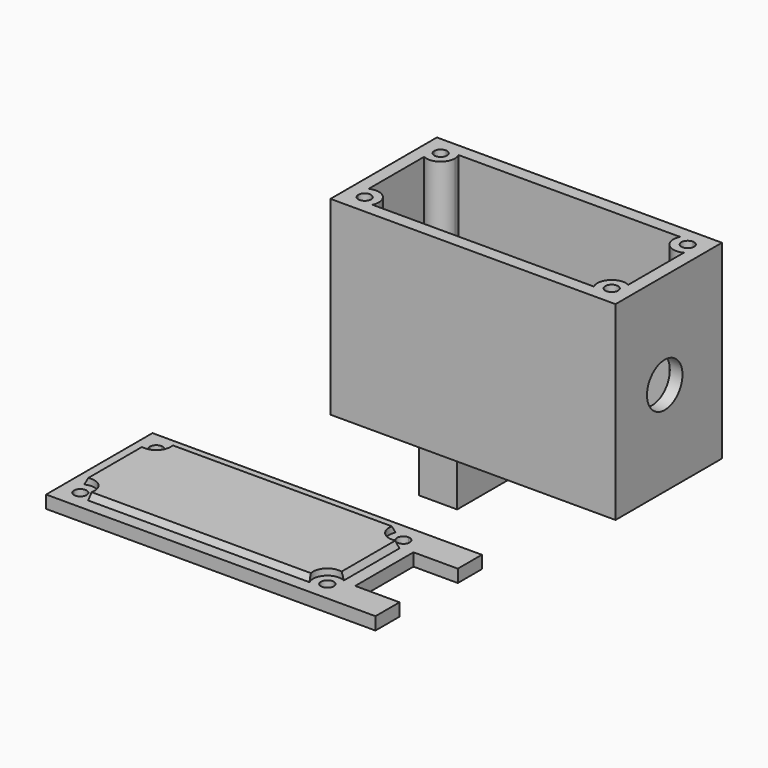
from build123d import *

# Parameters (mm, degrees)
F1_DEPTH = 30
F0_R     = 1
F2_DEPTH = 2
F3_DEPTH = 10
F4_DEPTH = 2
F5_DEPTH = 3
F6_SIZE2 = 0.99999
F6_SIZE  = 0.49999
F7_R     = 3.5
F8_DEPTH = 40
F0_W     = 7
F0_H     = 4.75
F9_DEPTH = 2


# Not quite as in the source:
# - a fillet or chamfer is up to 0.001 mm smaller than in the source, because OpenCascade refuses the exact size


with BuildPart() as f1:
    # F0 (on Top) → F1 (new body)
    with BuildSketch(Plane.XY):
        Polygon((-3, 1), (-1.2e-09, 1), (3, 1), (3, 3), (-3, 3), align=None)
        with BuildLine():
            Line((-7.9844355629, 1), (-3, 1))
            Line((-3, 1), (-3, 3))
            Line((-3, 3), (-13, 3))
            Line((-13, 3), (-13, -18))
            Line((-13, -18), (32, -18))
            Line((32, -18), (32, 3))
            Line((32, 3), (3, 3))
            Line((3, 3), (3, 1))
            Line((3, 1), (26.9844355629, 1))
            ThreePointArc((26.9844355629, 1), (29.5135562367, 2.1906072199), (31.25, 0))
            ThreePointArc((31.25, 0), (30.9121323176, -1.1858541226), (30, -2.0155644371))
            Line((30, -2.0155644371), (30, -12.9844355629))
            ThreePointArc((30, -12.9844355629), (30.9121323176, -13.8141458774), (31.25, -15))
            ThreePointArc((31.25, -15), (29.5135562367, -17.1906072199), (26.9844355629, -16))
            Line((26.9844355629, -16), (-7.9852204443, -16))
            ThreePointArc((-7.9852204443, -16), (-11.592084853, -16.5906804835), (-11, -12.9840463431))
            Line((-11, -12.9840463431), (-11, -2.0155644371))
            ThreePointArc((-11, -2.0155644371), (-11.5909902577, 1.5909902577), (-7.9844355629, 1))
        make_face()
        with BuildLine():
            ThreePointArc((-7.75, 0), (-7.8093927801, 0.5135562367), (-7.9844355629, 1))
            Line((-7.9844355629, 1), (-10, 1))
            ThreePointArc((-10, 1), (-9.2928932188, 0.7071067812), (-9, 0))
            ThreePointArc((-9, 0), (-10, -1), (-11, 0))
            Line((-11, 0), (-11, -2.0155644371))
            ThreePointArc((-11, -2.0155644371), (-8.8141458774, -1.9121323176), (-7.75, 0))
        make_face()
        with BuildLine():
            Line((-10, 1), (-7.9844355629, 1))
            ThreePointArc((-7.9844355629, 1), (-11.5909902577, 1.5909902577), (-11, -2.0155644371))
            Line((-11, -2.0155644371), (-11, 0))
            Line((-11, 0), (-11, 1))
            Line((-11, 1), (-10, 1))
        make_face()
        with BuildLine():
            ThreePointArc((31.25, 0), (29.5135562367, 2.1906072199), (26.9844355629, 1))
            Line((26.9844355629, 1), (29, 1))
            Line((29, 1), (30, 1))
            Line((30, 1), (30, 0))
            Line((30, 0), (30, -2.0155644371))
            ThreePointArc((30, -2.0155644371), (30.9121323176, -1.1858541226), (31.25, 0))
        make_face()
        with BuildLine():
            Line((29, 1), (26.9844355629, 1))
            ThreePointArc((26.9844355629, 1), (27.4090097423, -1.5909902577), (30, -2.0155644371))
            Line((30, -2.0155644371), (30, 0))
            ThreePointArc((30, 0), (28.2928932188, -0.7071067812), (29, 1))
        make_face()
        with BuildLine():
            Line((30, 1), (29, 1))
            ThreePointArc((29, 1), (29.7071067812, 0.7071067812), (30, 0))
            Line((30, 0), (30, 1))
        make_face()
        with BuildLine():
            ThreePointArc((-11, 0), (-10.7071067812, 0.7071067812), (-10, 1))
            Line((-10, 1), (-11, 1))
            Line((-11, 1), (-11, 0))
        make_face()
        with BuildLine():
            ThreePointArc((-10.0007848814, -16), (-10.6937450327, -15.7209758864), (-11, -15.0396124575))
            Line((-11, -15.0396124575), (-11, -16))
            Line((-11, -16), (-10.0007848814, -16))
        make_face()
        with BuildLine():
            Line((-11, -14.9603875425), (-11, -12.9840463431))
            ThreePointArc((-11, -12.9840463431), (-11.592084853, -16.5906804835), (-7.9852204443, -16))
            Line((-7.9852204443, -16), (-10.0007848814, -16))
            Line((-10.0007848814, -16), (-11, -16))
            Line((-11, -16), (-11, -15.0396124575))
            ThreePointArc((-11, -15.0396124575), (-11.0007848814, -15), (-11, -14.9603875425))
        make_face()
        with BuildLine():
            ThreePointArc((-7.7507848814, -15), (-8.8145585153, -13.0880985882), (-11, -12.9840463431))
            Line((-11, -12.9840463431), (-11, -14.9603875425))
            ThreePointArc((-11, -14.9603875425), (-9.9809747651, -14.0001962396), (-9.0007848814, -15))
            ThreePointArc((-9.0007848814, -15), (-9.2936781002, -15.7071067812), (-10.0007848814, -16))
            Line((-10.0007848814, -16), (-7.9852204443, -16))
            ThreePointArc((-7.9852204443, -16), (-7.8101776616, -15.5135562367), (-7.7507848814, -15))
        make_face()
        with BuildLine():
            Line((30, -16), (30, -15))
            ThreePointArc((30, -15), (29.7071067812, -15.7071067812), (29, -16))
            Line((29, -16), (30, -16))
        make_face()
        with BuildLine():
            Line((30, -15), (30, -12.9844355629))
            ThreePointArc((30, -12.9844355629), (27.4090097423, -13.4090097423), (26.9844355629, -16))
            Line((26.9844355629, -16), (29, -16))
            ThreePointArc((29, -16), (28.2928932188, -14.2928932188), (30, -15))
        make_face()
        with BuildLine():
            ThreePointArc((31.25, -15), (30.9121323176, -13.8141458774), (30, -12.9844355629))
            Line((30, -12.9844355629), (30, -15))
            Line((30, -15), (30, -16))
            Line((30, -16), (29, -16))
            Line((29, -16), (26.9844355629, -16))
            ThreePointArc((26.9844355629, -16), (29.5135562367, -17.1906072199), (31.25, -15))
        make_face()
    extrude(amount=F1_DEPTH)

    # F0 (on Top) → F2 (join)
    with BuildSketch(Plane.XY):
        with BuildLine():
            Line((-3, -13), (-3, 1))
            Line((-3, 1), (-7.9844355629, 1))
            ThreePointArc((-7.9844355629, 1), (-7.8093927801, 0.5135562367), (-7.75, 0))
            ThreePointArc((-7.75, 0), (-8.8141458774, -1.9121323176), (-11, -2.0155644371))
            Line((-11, -2.0155644371), (-11, -12.9840463431))
            ThreePointArc((-11, -12.9840463431), (-8.8145585153, -13.0880985882), (-7.7507848814, -15))
            ThreePointArc((-7.7507848814, -15), (-7.8101776616, -15.5135562367), (-7.9852204443, -16))
            Line((-7.9852204443, -16), (26.9844355629, -16))
            ThreePointArc((26.9844355629, -16), (27.4090097423, -13.4090097423), (30, -12.9844355629))
            Line((30, -12.9844355629), (30, -2.0155644371))
            ThreePointArc((30, -2.0155644371), (27.4090097423, -1.5909902577), (26.9844355629, 1))
            Line((26.9844355629, 1), (3, 1))
            Line((3, 1), (3, -13))
            Line((3, -13), (-3, -13))
        make_face()
        Polygon((3, 1), (-1.2e-09, 1), (-3, 1), (-3, -13), (3, -13), align=None)
        with Locations((0, -10)):
            Circle(F0_R, mode=Mode.SUBTRACT)
        with BuildLine():
            ThreePointArc((-1.2e-09, 1), (0.7071067808, 0.7071067816), (1, 0))
            ThreePointArc((1, 0), (-0.7071067808, -0.7071067816), (-1.2e-09, 1))
        make_face(mode=Mode.SUBTRACT)
        with BuildLine():
            ThreePointArc((-1.2e-09, 1), (-0.7071067808, -0.7071067816), (1, 0))
            ThreePointArc((1, 0), (0.7071067808, 0.7071067816), (-1.2e-09, 1))
        make_face()
        with BuildLine():
            ThreePointArc((-9, 0), (-9.2928932188, 0.7071067812), (-10, 1))
            ThreePointArc((-10, 1), (-10.7071067812, 0.7071067812), (-11, 0))
            ThreePointArc((-11, 0), (-10, -1), (-9, 0))
        make_face()
        with BuildLine():
            ThreePointArc((30, 0), (29.7071067812, 0.7071067812), (29, 1))
            ThreePointArc((29, 1), (28.2928932188, -0.7071067812), (30, 0))
        make_face()
        with BuildLine():
            ThreePointArc((29, -16), (29.7071067812, -15.7071067812), (30, -15))
            ThreePointArc((30, -15), (28.2928932188, -14.2928932188), (29, -16))
        make_face()
        with Locations((0, -10)):
            Circle(F0_R)
        with BuildLine():
            ThreePointArc((-9.0007848814, -15), (-9.9809747651, -14.0001962396), (-11, -14.9603875425))
            Line((-11, -14.9603875425), (-11, -15.0396124575))
            ThreePointArc((-11, -15.0396124575), (-10.6937450327, -15.7209758864), (-10.0007848814, -16))
            ThreePointArc((-10.0007848814, -16), (-9.2936781002, -15.7071067812), (-9.0007848814, -15))
        make_face()
        with BuildLine():
            Line((-11, -15.0396124575), (-11, -14.9603875425))
            ThreePointArc((-11, -14.9603875425), (-11.0007848814, -15), (-11, -15.0396124575))
        make_face()
    extrude(amount=F2_DEPTH)

    # F0 (on Top) → F3 (join)
    with BuildSketch(Plane.XY):
        Polygon((3, 1), (-1.2e-09, 1), (-3, 1), (-3, -13), (3, -13), align=None)
        with Locations((0, -10)):
            Circle(F0_R, mode=Mode.SUBTRACT)
        with BuildLine():
            ThreePointArc((-1.2e-09, 1), (0.7071067808, 0.7071067816), (1, 0))
            ThreePointArc((1, 0), (-0.7071067808, -0.7071067816), (-1.2e-09, 1))
        make_face(mode=Mode.SUBTRACT)
        Polygon((-3, 1), (-1.2e-09, 1), (3, 1), (3, 3), (-3, 3), align=None)
    extrude(amount=-F3_DEPTH)

    # F7 (on Right) → F8 (cut)
    with BuildSketch(Plane.YZ):
        with Locations((-8.2862954587, 14.8329315707)):
            Circle(F7_R)
    extrude(amount=F8_DEPTH, mode=Mode.SUBTRACT)


with BuildPart() as f4:
    # F0 (on Top) → F4 (new body)
    with BuildSketch(Plane.XY):
        with BuildLine():
            Line((-19.6516566587, -40.5400313383), (-14.6672210958, -40.5400313383))
            Line((-14.6672210958, -40.5400313383), (-14.6672210958, -38.5400313383))
            Line((-14.6672210958, -38.5400313383), (-24.6672210958, -38.5400313383))
            Line((-24.6672210958, -38.5400313383), (-24.6672210958, -59.5400313383))
            Line((-24.6672210958, -59.5400313383), (20.3327789042, -59.5400313383))
            Line((20.3327789042, -59.5400313383), (20.3327789042, -54.7900313383))
            Line((20.3327789042, -54.7900313383), (20.3327789042, -43.2900313383))
            Line((20.3327789042, -43.2900313383), (20.3327789042, -38.5400313383))
            Line((20.3327789042, -38.5400313383), (-8.6672210958, -38.5400313383))
            Line((-8.6672210958, -38.5400313383), (-8.6672210958, -40.5400313383))
            Line((-8.6672210958, -40.5400313383), (15.3172144672, -40.5400313383))
            ThreePointArc((15.3172144672, -40.5400313383), (17.846335141, -39.3494241184), (19.5827789042, -41.5400313383))
            ThreePointArc((19.5827789042, -41.5400313383), (19.2449112218, -42.7258854608), (18.3327789042, -43.5555957754))
            Line((18.3327789042, -43.5555957754), (18.3327789042, -54.5244669012))
            ThreePointArc((18.3327789042, -54.5244669012), (19.2449112218, -55.3541772157), (19.5827789042, -56.5400313383))
            ThreePointArc((19.5827789042, -56.5400313383), (17.846335141, -58.7306385581), (15.3172144672, -57.5400313383))
            Line((15.3172144672, -57.5400313383), (-19.6524415401, -57.5400313383))
            ThreePointArc((-19.6524415401, -57.5400313383), (-23.2593059487, -58.1307118218), (-22.6672210958, -54.5240776814))
            Line((-22.6672210958, -54.5240776814), (-22.6672210958, -43.5555957754))
            ThreePointArc((-22.6672210958, -43.5555957754), (-23.2582113534, -39.9490410806), (-19.6516566587, -40.5400313383))
        make_face()
        Polygon((-14.6672210958, -40.5400313383), (-11.6672210958, -40.5400313383), (-8.6672210958, -40.5400313383), (-8.6672210958, -38.5400313383), (-14.6672210958, -38.5400313383), align=None)
        with BuildLine():
            ThreePointArc((-19.4172210958, -41.5400313383), (-19.4766138759, -41.0264751015), (-19.6516566587, -40.5400313383))
            Line((-19.6516566587, -40.5400313383), (-21.6672210958, -40.5400313383))
            ThreePointArc((-21.6672210958, -40.5400313383), (-20.9601143146, -40.8329245571), (-20.6672210958, -41.5400313383))
            ThreePointArc((-20.6672210958, -41.5400313383), (-21.6672210958, -42.5400313383), (-22.6672210958, -41.5400313383))
            Line((-22.6672210958, -41.5400313383), (-22.6672210958, -43.5555957754))
            ThreePointArc((-22.6672210958, -43.5555957754), (-20.4813669732, -43.4521636559), (-19.4172210958, -41.5400313383))
        make_face()
        with BuildLine():
            ThreePointArc((-19.4180059772, -56.5400313383), (-20.4817796111, -54.6281299265), (-22.6672210958, -54.5240776814))
            Line((-22.6672210958, -54.5240776814), (-22.6672210958, -56.5004188808))
            ThreePointArc((-22.6672210958, -56.5004188808), (-21.6481958609, -55.5402275779), (-20.6680059772, -56.5400313383))
            ThreePointArc((-20.6680059772, -56.5400313383), (-20.960899196, -57.2471381195), (-21.6680059772, -57.5400313383))
            Line((-21.6680059772, -57.5400313383), (-19.6524415401, -57.5400313383))
            ThreePointArc((-19.6524415401, -57.5400313383), (-19.4773987573, -57.053587575), (-19.4180059772, -56.5400313383))
        make_face()
        with BuildLine():
            ThreePointArc((19.5827789042, -41.5400313383), (17.846335141, -39.3494241184), (15.3172144672, -40.5400313383))
            Line((15.3172144672, -40.5400313383), (17.332778938, -40.5400313383))
            Line((17.332778938, -40.5400313383), (18.3327789042, -40.5400313383))
            Line((18.3327789042, -40.5400313383), (18.3327789042, -41.5400313383))
            Line((18.3327789042, -41.5400313383), (18.3327789042, -43.5555957754))
            ThreePointArc((18.3327789042, -43.5555957754), (19.2449112218, -42.7258854608), (19.5827789042, -41.5400313383))
        make_face()
        with BuildLine():
            Line((17.332778938, -40.5400313383), (15.3172144672, -40.5400313383))
            ThreePointArc((15.3172144672, -40.5400313383), (15.7417886466, -43.1310215959), (18.3327789042, -43.5555957754))
            Line((18.3327789042, -43.5555957754), (18.3327789042, -41.5400313383))
            ThreePointArc((18.3327789042, -41.5400313383), (16.6256721111, -42.2471381075), (17.332778938, -40.5400313383))
        make_face()
        with BuildLine():
            Line((18.3327789042, -56.5400313383), (18.3327789042, -54.5244669012))
            ThreePointArc((18.3327789042, -54.5244669012), (15.7417886466, -54.9490410806), (15.3172144672, -57.5400313383))
            Line((15.3172144672, -57.5400313383), (17.3327789042, -57.5400313383))
            ThreePointArc((17.3327789042, -57.5400313383), (16.6256721231, -55.8329245571), (18.3327789042, -56.5400313383))
        make_face()
        with BuildLine():
            Line((18.3327789042, -57.5400313383), (18.3327789042, -56.5400313383))
            ThreePointArc((18.3327789042, -56.5400313383), (18.0398856854, -57.2471381195), (17.3327789042, -57.5400313383))
            Line((17.3327789042, -57.5400313383), (18.3327789042, -57.5400313383))
        make_face()
        with BuildLine():
            ThreePointArc((19.5827789042, -56.5400313383), (19.2449112218, -55.3541772157), (18.3327789042, -54.5244669012))
            Line((18.3327789042, -54.5244669012), (18.3327789042, -56.5400313383))
            Line((18.3327789042, -56.5400313383), (18.3327789042, -57.5400313383))
            Line((18.3327789042, -57.5400313383), (17.3327789042, -57.5400313383))
            Line((17.3327789042, -57.5400313383), (15.3172144672, -57.5400313383))
            ThreePointArc((15.3172144672, -57.5400313383), (17.846335141, -58.7306385581), (19.5827789042, -56.5400313383))
        make_face()
        with BuildLine():
            Line((-22.6672210958, -56.5004188808), (-22.6672210958, -54.5240776814))
            ThreePointArc((-22.6672210958, -54.5240776814), (-23.2593059487, -58.1307118218), (-19.6524415401, -57.5400313383))
            Line((-19.6524415401, -57.5400313383), (-21.6680059772, -57.5400313383))
            Line((-21.6680059772, -57.5400313383), (-22.6672210958, -57.5400313383))
            Line((-22.6672210958, -57.5400313383), (-22.6672210958, -56.5796437958))
            ThreePointArc((-22.6672210958, -56.5796437958), (-22.6680059772, -56.5400313383), (-22.6672210958, -56.5004188808))
        make_face()
        with BuildLine():
            Line((-21.6672210958, -40.5400313383), (-19.6516566587, -40.5400313383))
            ThreePointArc((-19.6516566587, -40.5400313383), (-23.2582113534, -39.9490410806), (-22.6672210958, -43.5555957754))
            Line((-22.6672210958, -43.5555957754), (-22.6672210958, -41.5400313383))
            Line((-22.6672210958, -41.5400313383), (-22.6672210958, -40.5400313383))
            Line((-22.6672210958, -40.5400313383), (-21.6672210958, -40.5400313383))
        make_face()
        with BuildLine():
            ThreePointArc((-22.6672210958, -41.5400313383), (-22.3743278769, -40.8329245571), (-21.6672210958, -40.5400313383))
            Line((-21.6672210958, -40.5400313383), (-22.6672210958, -40.5400313383))
            Line((-22.6672210958, -40.5400313383), (-22.6672210958, -41.5400313383))
        make_face()
        with BuildLine():
            ThreePointArc((-21.6680059772, -57.5400313383), (-22.3609661284, -57.2610072247), (-22.6672210958, -56.5796437958))
            Line((-22.6672210958, -56.5796437958), (-22.6672210958, -57.5400313383))
            Line((-22.6672210958, -57.5400313383), (-21.6680059772, -57.5400313383))
        make_face()
        with BuildLine():
            Line((18.3327789042, -40.5400313383), (17.332778938, -40.5400313383))
            ThreePointArc((17.332778938, -40.5400313383), (18.0398856974, -40.832924569), (18.3327789042, -41.5400313383))
            Line((18.3327789042, -41.5400313383), (18.3327789042, -40.5400313383))
        make_face()
    extrude(amount=F4_DEPTH)

    # F0 (on Top) → F5 (join)
    with BuildSketch(Plane.XY):
        with BuildLine():
            Line((-14.6672210958, -54.5400313383), (-14.6672210958, -40.5400313383))
            Line((-14.6672210958, -40.5400313383), (-19.6516566587, -40.5400313383))
            ThreePointArc((-19.6516566587, -40.5400313383), (-19.4766138759, -41.0264751015), (-19.4172210958, -41.5400313383))
            ThreePointArc((-19.4172210958, -41.5400313383), (-20.4813669732, -43.4521636559), (-22.6672210958, -43.5555957754))
            Line((-22.6672210958, -43.5555957754), (-22.6672210958, -54.5240776814))
            ThreePointArc((-22.6672210958, -54.5240776814), (-20.4817796111, -54.6281299265), (-19.4180059772, -56.5400313383))
            ThreePointArc((-19.4180059772, -56.5400313383), (-19.4773987573, -57.053587575), (-19.6524415401, -57.5400313383))
            Line((-19.6524415401, -57.5400313383), (15.3172144672, -57.5400313383))
            ThreePointArc((15.3172144672, -57.5400313383), (15.7417886466, -54.9490410806), (18.3327789042, -54.5244669012))
            Line((18.3327789042, -54.5244669012), (18.3327789042, -43.5555957754))
            ThreePointArc((18.3327789042, -43.5555957754), (15.7417886466, -43.1310215959), (15.3172144672, -40.5400313383))
            Line((15.3172144672, -40.5400313383), (-8.6672210958, -40.5400313383))
            Line((-8.6672210958, -40.5400313383), (-8.6672210958, -54.5400313383))
            Line((-8.6672210958, -54.5400313383), (-14.6672210958, -54.5400313383))
        make_face()
        Polygon((-8.6672210958, -40.5400313383), (-11.6672210958, -40.5400313383), (-14.6672210958, -40.5400313383), (-14.6672210958, -54.5400313383), (-8.6672210958, -54.5400313383), align=None)
        with Locations((-11.6672210958, -51.5400313383)):
            Circle(F0_R, mode=Mode.SUBTRACT)
        with BuildLine():
            ThreePointArc((-11.6672210958, -40.5400313383), (-10.9601143146, -40.8329245571), (-10.6672210958, -41.5400313383))
            ThreePointArc((-10.6672210958, -41.5400313383), (-12.3743278769, -42.2471381195), (-11.6672210958, -40.5400313383))
        make_face(mode=Mode.SUBTRACT)
        with BuildLine():
            ThreePointArc((-11.6672210958, -40.5400313383), (-12.3743278769, -42.2471381195), (-10.6672210958, -41.5400313383))
            ThreePointArc((-10.6672210958, -41.5400313383), (-10.9601143146, -40.8329245571), (-11.6672210958, -40.5400313383))
        make_face()
        with Locations((-11.6672210958, -51.5400313383)):
            Circle(F0_R)
    extrude(amount=F5_DEPTH)

    # F6 (size 0.5 and 1 in the source; OpenCascade refuses exactly that, so slightly less here)
    f6_edges = [f4.edges().sort_by_distance(p)[0] for p in [
        (-2.167614, -57.540031, 3),
        (-22.667221, -49.039837, 3),
        (-2.167221, -40.540031, 3),
        (18.332779, -49.040031, 3),
    ]]
    f6_side = f4.faces().sort_by_distance((-2.167284, -49.040056, 3))[0]
    chamfer(f6_edges, length=F6_SIZE, length2=F6_SIZE2, reference=f6_side)

    # F0 (on Top) → F9 (join)
    with BuildSketch(Plane.XY):
        with Locations((23.8327789042, -40.9150313383)):
            Rectangle(F0_W, F0_H)
        with Locations((23.8327789042, -57.1650313383)):
            Rectangle(F0_W, F0_H)
    extrude(amount=F9_DEPTH)


solid = Compound([f1.part, f4.part])
